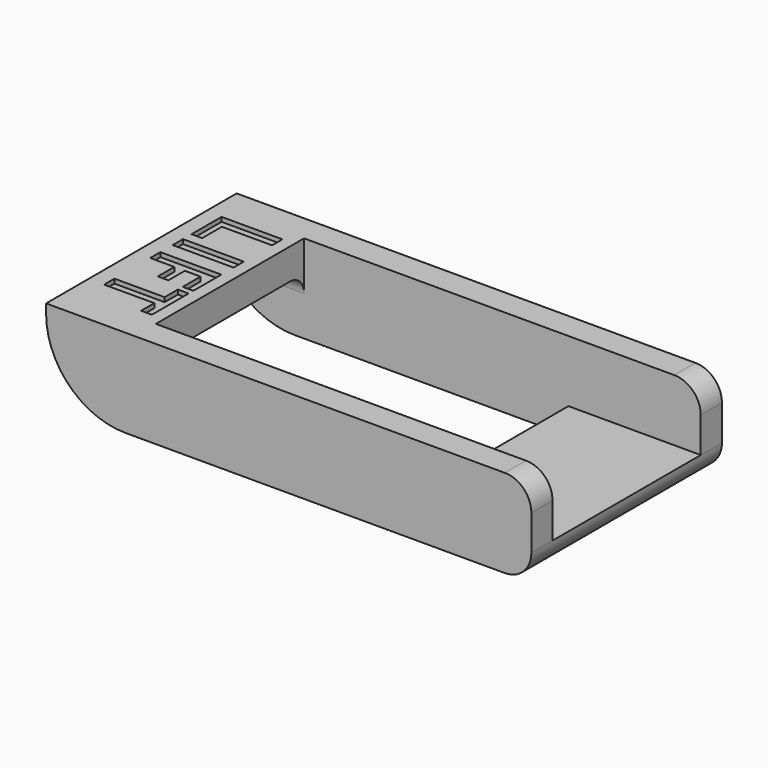
from build123d import *

# Parameters (mm, degrees)
F0_W         = 15
F0_H         = 21
F1_DEPTH     = 3
F2_DEPTH     = 10
F3_W         = 10.0380332768
F3_H         = 23.7995406166
F3_H_2       = 3
F4_DEPTH     = 3.5
F5_R         = 2.99999
F6_R         = 2
F7_T1_DEPTH  = 48
F7_T3_DEPTH  = 48
F8_R         = 2
F9_TEXT_SIZE = 9.6669435843
F10_DEPTH    = 0.5


# Not quite as in the source:
# - a fillet or chamfer that OpenCascade refuses, or shapes differently, is made with other operations: its cross-section is extruded or revolved along the edge and cut away or added
# - a fillet or chamfer is up to 0.001 mm smaller than in the source, because OpenCascade refuses the exact size
# - Text() gives the source's letters only with a copy of the font that has no kerning and outlines rounded to 1/6400 em; it was checked with that copy


with BuildPart() as f1:
    # F0 (on Top) → F1 (new body)
    with BuildSketch(Plane.XY):
        with Locations((20, 0)):
            Rectangle(F0_W, F0_H)
    extrude(amount=F1_DEPTH)

    # F0 (on Top) → F2 (join)
    with BuildSketch(Plane.XY):
        Polygon((27.5, -13.5), (27.5, -10.5), (12.5, -10.5), (-7.5, -10.5), (-27.5, -10.5), (-27.5, -13.5), align=None)
        Polygon((12.5, 10.5), (27.5, 10.5), (27.5, 13.5), (-27.5, 13.5), (-27.5, 10.5), (-7.5, 10.5), align=None)
    extrude(amount=F2_DEPTH)

    # F3 (on face) → F4 (join)
    with BuildSketch(Plane.XY.offset(10)):
        with Locations((-22.4809833616, -1.3997703083)):
            Rectangle(F3_W, F3_H)
        with Locations((-22.4809833616, 12)):
            Rectangle(F3_W, F3_H_2)
    extrude(amount=-F4_DEPTH)

    # F5 (radius 3 in the source; OpenCascade refuses exactly that, so slightly less here)
    f5_edges = [f1.edges().sort_by_distance(p)[0] for p in [
        (27.5, 0, 0),
        (27.5, -12, 10),
        (27.5, 12, 10),
    ]]
    fillet(f5_edges, radius=F5_R)

    # F6
    f6_edges = [f1.edges().sort_by_distance(p)[0] for p in [
        (-27.5, 0, 6.5),
    ]]
    fillet(f6_edges, radius=F6_R)

    # F7: fillet of radius 9 on 2 edges, made by hand

    # F7_s2 → F7_t1 (cut)
    with BuildSketch(Plane.XZ.offset(-36)):
        with BuildLine():
            ThreePointArc((-27.5, 9), (-24.8639610307, 2.6360389693), (-18.5, 0))
            Line((-18.5, 0), (-27.5, 0))
            Line((-27.5, 0), (-27.5, 9))
        make_face()
    extrude(amount=F7_T1_DEPTH, mode=Mode.SUBTRACT)

    # F7_s4 → F7_t3 (cut)
    with BuildSketch(Plane.XZ.offset(-12)):
        with BuildLine():
            ThreePointArc((-27.5, 9), (-24.8639610307, 2.6360389693), (-18.5, 0))
            Line((-18.5, 0), (-27.5, 0))
            Line((-27.5, 0), (-27.5, 9))
        make_face()
    extrude(amount=F7_T3_DEPTH, mode=Mode.SUBTRACT)

    # F8
    f8_edges = [f1.edges().sort_by_distance(p)[0] for p in [
        (-21.480983, 10.5, 6.5),
        (-21.480983, -10.5, 6.5),
    ]]
    fillet(f8_edges, radius=F8_R)

    # F9 (on face) → F10 (cut)
    with BuildSketch(Plane.XY.offset(10)):
        with Locations(Location((-25.7357304951, 10.0221510639), (0, 0, -90))):
            Text('LIFT', F9_TEXT_SIZE, font='Open Sans', font_style=FontStyle.BOLD, text_align=(TextAlign.LEFT, TextAlign.BOTTOM))
    extrude(amount=-F10_DEPTH, mode=Mode.SUBTRACT)


solid = f1.part
